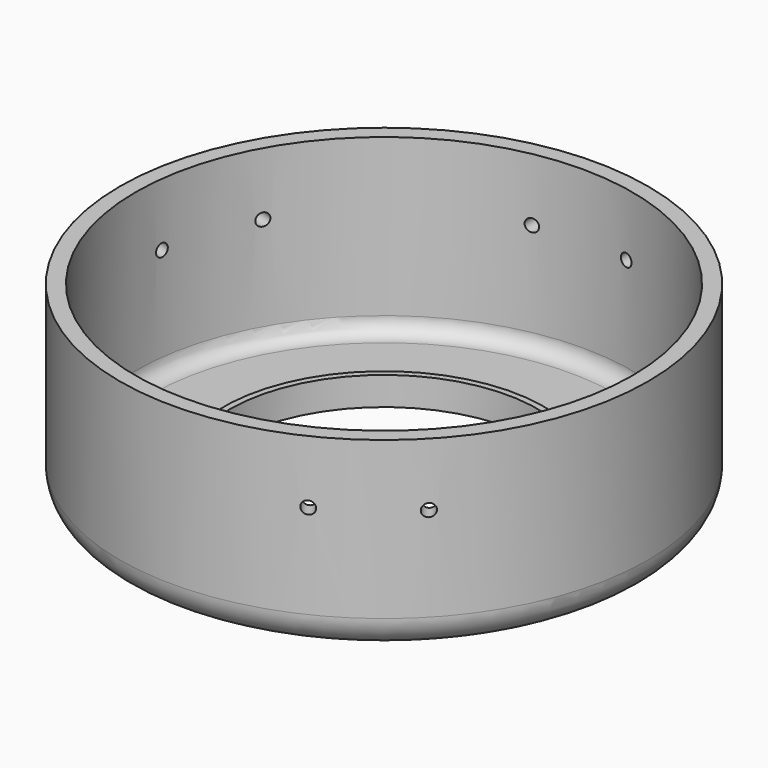
from build123d import *

# Parameters (mm, degrees)
F0_R            = 42
F0_R_2          = 25.5
F0_R_3          = 24.5
F1_DEPTH        = 30
F2_R            = 5
F3_T            = -2.5
F4_R            = 1
F5_DEPTH        = 100
F5_COPIES_COUNT = 3
F5_COPIES_ANGLE = 288
F6_DEPTH        = 25
F7_DEPTH        = 4.5
F8_SIZE         = 1.99999
F9_W            = 2.5
F9_H            = 25
F10_ANGLE       = 68.1766396911


# Not quite as in the source:
# - a fillet or chamfer is up to 0.001 mm smaller than in the source, because OpenCascade refuses the exact size
# - a pattern or mirror of a feature is missing from the dataset's text; its kind, count and spacing are read off the source's solid


with BuildPart() as f1:
    # F0 (on Top) → F1 (new body)
    with BuildSketch(Plane.XY):
        Circle(F0_R)
        Circle(F0_R_2, mode=Mode.SUBTRACT)
        Circle(F0_R_2)
        Circle(F0_R_3, mode=Mode.SUBTRACT)
        Circle(F0_R_3)
    extrude(amount=F1_DEPTH)

    # F2
    f2_edges = [f1.edges().sort_by_distance(p)[0] for p in [
        (-42, 0, 0),
    ]]
    fillet(f2_edges, radius=F2_R)

    # F3
    f3_openings = [f1.faces().sort_by_distance(p)[0] for p in [
        (0, 0, 30),
    ]]
    offset(amount=F3_T, openings=f3_openings)

    # F4 (on Front) → F5 (cut)
    with BuildSketch(Plane.XZ):
        with Locations((-7.5, 20)):
            Circle(F4_R)
        with Locations((7.5, 20)):
            Circle(F4_R)
    f5 = extrude(amount=-F5_DEPTH, mode=Mode.SUBTRACT)

    # F5_copies: F5 ×3 about axis
    f5_copies_axis = Axis((0, 0, 0), (0, 0, -1))
    for i in range(1, F5_COPIES_COUNT):
        add(f5.rotate(f5_copies_axis, i * F5_COPIES_ANGLE / (F5_COPIES_COUNT - 1)), mode=Mode.SUBTRACT)

    # F0 (on Top) → F6 (cut)
    with BuildSketch(Plane.XY):
        Circle(F0_R_3)
    extrude(amount=F6_DEPTH, mode=Mode.SUBTRACT)

    # F0 (on Top) → F7 (join)
    with BuildSketch(Plane.XY):
        Circle(F0_R_2)
        Circle(F0_R_3, mode=Mode.SUBTRACT)
    extrude(amount=F7_DEPTH)

    # F8 (size 2 in the source; OpenCascade refuses exactly that, so slightly less here)
    f8_edges = [f1.edges().sort_by_distance(p)[0] for p in [
        (-25.5, 0, 2.5),
    ]]
    chamfer(f8_edges, length=F8_SIZE)

    # F9 (on Front) → F10 (revolve)
    with BuildSketch(Plane.XZ):
        with Locations((40.75, 17.5)):
            Rectangle(F9_W, F9_H)
        with Locations((-40.75, 17.5)):
            Rectangle(F9_W, F9_H)
    revolve(axis=Axis((0, 0, 30), (0, 0, 1)), revolution_arc=F10_ANGLE)


solid = f1.part
